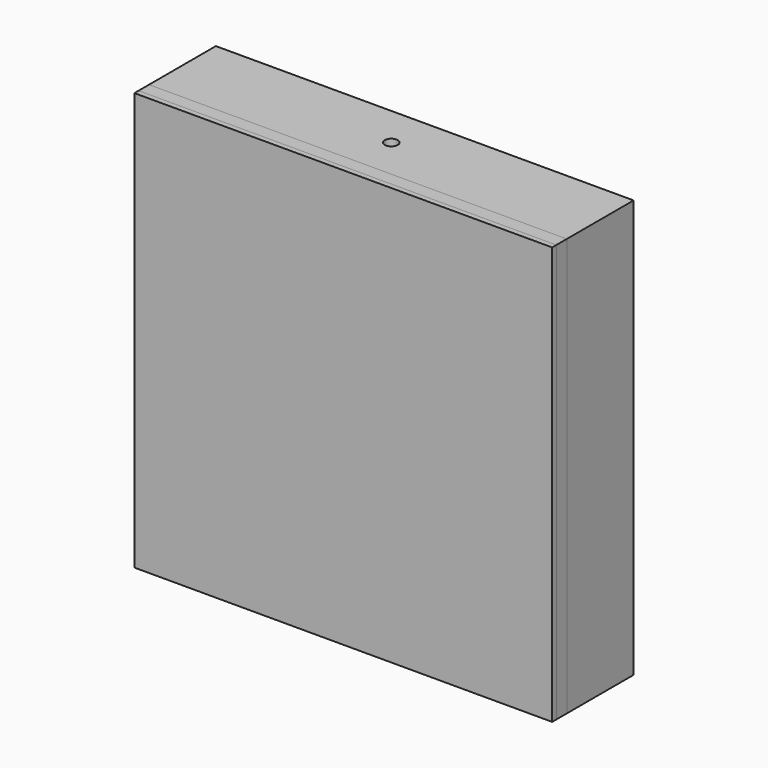
from build123d import *

# Parameters (mm, degrees)
F0_R     = 3.175
F0_W     = 12.7
F0_H     = 12.7
F1_DEPTH = 6.35
F2_DEPTH = 20.32
F3_R     = 1.5875
F4_DEPTH = 25.4
F5_W     = 101.6
F5_H     = 101.6
F5_R     = 3.175
F5_W_2   = 76.2
F5_H_2   = 76.2
F6_DEPTH = 3.175
F7_W     = 101.6
F7_H     = 101.6
F7_R     = 3.175
F7_W_2   = 76.2
F7_H_2   = 76.2
F8_DEPTH = 1.27


# Not quite as in the source:
# - a feature names something its author has since deleted; it is built from what else it names


with BuildPart() as f1:
    # F0 (on Front) → F1 (new body)
    with BuildSketch(Plane.XZ):
        Polygon((38.1, 38.1), (38.1, 0), (38.1, -38.1), (-38.1, -38.1), (-38.1, 0), (-38.1, 38.1), (-50.8, 38.1), (-50.8, -50.8), (50.8, -50.8), (50.8, 38.1), align=None)
        with Locations((-44.45, -44.45)):
            Circle(F0_R, mode=Mode.SUBTRACT)
        with Locations((44.45, -44.45)):
            Circle(F0_R, mode=Mode.SUBTRACT)
        Polygon((38.1, -38.1), (38.1, 0), (38.1, 38.1), (0, 38.1), (-38.1, 38.1), (-38.1, 0), (-38.1, -38.1), align=None)
        Polygon((0, 38.1), (38.1, 38.1), (38.1, 50.8), (-38.1, 50.8), (-38.1, 38.1), align=None)
        with Locations((-44.45, 44.45)):
            Rectangle(F0_W, F0_H)
        with Locations((-44.45, 44.45)):
            Circle(F0_R, mode=Mode.SUBTRACT)
        with Locations((44.45, 44.45)):
            Rectangle(F0_W, F0_H)
        with Locations((44.45, 44.45)):
            Circle(F0_R, mode=Mode.SUBTRACT)
    extrude(amount=F1_DEPTH)

    # F0 (on Front) → F2 (join)
    with BuildSketch(Plane.XZ):
        Polygon((38.1, 38.1), (38.1, 0), (38.1, -38.1), (-38.1, -38.1), (-38.1, 0), (-38.1, 38.1), (-50.8, 38.1), (-50.8, -50.8), (50.8, -50.8), (50.8, 38.1), align=None)
        with Locations((-44.45, -44.45)):
            Circle(F0_R, mode=Mode.SUBTRACT)
        with Locations((44.45, -44.45)):
            Circle(F0_R, mode=Mode.SUBTRACT)
        Polygon((0, 38.1), (38.1, 38.1), (38.1, 50.8), (-38.1, 50.8), (-38.1, 38.1), align=None)
        with Locations((44.45, 44.45)):
            Rectangle(F0_W, F0_H)
        with Locations((44.45, 44.45)):
            Circle(F0_R, mode=Mode.SUBTRACT)
        with Locations((-44.45, 44.45)):
            Rectangle(F0_W, F0_H)
        with Locations((-44.45, 44.45)):
            Circle(F0_R, mode=Mode.SUBTRACT)
    extrude(amount=F2_DEPTH)

    # F3 (on face) → F4 (cut)
    with BuildSketch(Plane.XY.offset(50.8)):
        with Locations((0, -10.16)):
            Circle(F3_R)
    extrude(amount=-F4_DEPTH, mode=Mode.SUBTRACT)


with BuildPart() as f6:
    # F5 (on face) → F6 (new body)
    with BuildSketch(Plane.XZ.offset(20.32)):
        Rectangle(F5_W, F5_H)
        with Locations((-44.45, -44.45)):
            Circle(F5_R, mode=Mode.SUBTRACT)
        Rectangle(F5_W_2, F5_H_2, mode=Mode.SUBTRACT)
        with Locations((44.45, -44.45)):
            Circle(F5_R, mode=Mode.SUBTRACT)
        with Locations((-44.45, 44.45)):
            Circle(F5_R, mode=Mode.SUBTRACT)
        with Locations((44.45, 44.45)):
            Circle(F5_R, mode=Mode.SUBTRACT)
    extrude(amount=F6_DEPTH)


with BuildPart() as f8:
    # F7 (on face) → F8 (new body)
    with BuildSketch(Plane.XZ.offset(23.495)):
        Rectangle(F7_W, F7_H)
        with Locations((-44.45, -44.45)):
            Circle(F7_R, mode=Mode.SUBTRACT)
        Rectangle(F7_W_2, F7_H_2, mode=Mode.SUBTRACT)
        with Locations((44.45, -44.45)):
            Circle(F7_R, mode=Mode.SUBTRACT)
        with Locations((-44.45, 44.45)):
            Circle(F7_R, mode=Mode.SUBTRACT)
        with Locations((44.45, 44.45)):
            Circle(F7_R, mode=Mode.SUBTRACT)
        with Locations((-44.45, -44.45)):
            Circle(F7_R)
        Rectangle(F7_W_2, F7_H_2)
        with Locations((44.45, -44.45)):
            Circle(F7_R)
        with Locations((-44.45, 44.45)):
            Circle(F7_R)
        with Locations((44.45, 44.45)):
            Circle(F7_R)
    extrude(amount=F8_DEPTH)


solid = Compound([f1.part, f6.part, f8.part])
